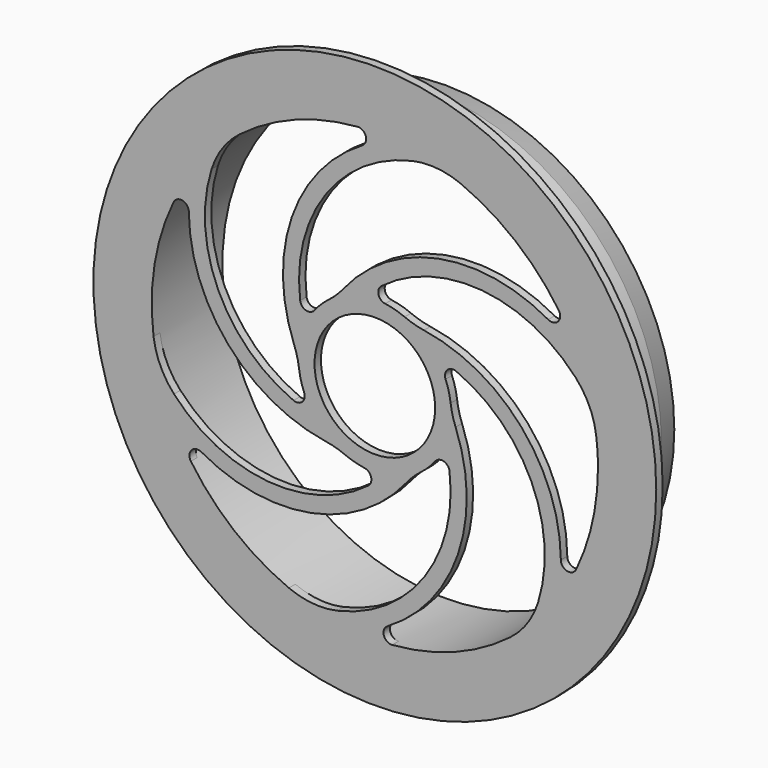
from build123d import *

# Parameters (mm, degrees)
F0_R            = 29.25
F0_R_2          = 27.75
F1_DEPTH        = 10
F2_R            = 35
F2_R_2          = 27.75
F3_DEPTH        = 1
F4_R            = 9.5
F4_R_2          = 7.5
F5_DEPTH        = 1
F7_DEPTH        = 1
F7_COPIES_COUNT = 6
F8_R            = 1
F9_T1_DEPTH     = 1
F10_SIZE2       = 0.8038475773
F10_SIZE        = 3


# Not quite as in the source:
# - a fillet or chamfer that OpenCascade refuses, or shapes differently, is made with other operations: its cross-section is extruded or revolved along the edge and cut away or added
# - a pattern or mirror of a feature is missing from the dataset's text; its kind, count and spacing are read off the source's solid


with BuildPart() as f1:
    # F0 (on Front) → F1 (new body)
    with BuildSketch(Plane.XZ):
        Circle(F0_R)
        Circle(F0_R_2, mode=Mode.SUBTRACT)
    extrude(amount=-F1_DEPTH)

    # F2 (on face) → F3 (join)
    with BuildSketch(Plane.XZ):
        Circle(F2_R)
        Circle(F2_R_2, mode=Mode.SUBTRACT)
    extrude(amount=F3_DEPTH)



with BuildPart() as f5:
    # F4 (on face) → F5 (new body)
    with BuildSketch(Plane.XZ.offset(1)):
        Circle(F4_R)
        Circle(F4_R_2, mode=Mode.SUBTRACT)
    extrude(amount=-F5_DEPTH)


with BuildPart() as f1_1:
    add(f1.part)

    add(f5.part)  # F7 merges F5
    # F6 (on face) → F7 (join)
    with BuildSketch(Plane.XZ.offset(1)):
        with BuildLine():
            ThreePointArc((8.0310171435, 26.562478492), (5.3050841985, 27.2381824219), (2.5248144723, 27.6349020603))
            ThreePointArc((2.5248144723, 27.6349020603), (-9.7684943804, 16.550468737), (-9.5, 0))
            Line((-9.5, 0), (-8.1966003247, 2.0236510077))
            ThreePointArc((-8.1966003247, 2.0236510077), (-6.4433975316, 18.4993570083), (8.0310171435, 26.562478492))
        make_face()
    f7 = extrude(amount=-F7_DEPTH)

    # F7_copies: F7 ×6 about axis
    f7_copies_axis = Axis((0, 0, 0), (0, 1, 0))
    for i in range(1, F7_COPIES_COUNT):
        add(f7.rotate(f7_copies_axis, i * 360 / F7_COPIES_COUNT))

    # F8
    f8_edges = [f1_1.edges().sort_by_distance(p)[0] for p in [
        (-8.754714, -0.5, 3.688493),
        (27.75, -0.5, 0),
        (25.194934, -0.5, 11.630898),
        (-1.183028, -0.5, 9.426051),
        (22.67012, -0.5, -16.004005),
        (7.571686, -0.5, 5.737558),
        (-2.524814, -0.5, -27.634902),
        (8.754714, -0.5, -3.688493),
        (-25.194934, -0.5, -11.630898),
        (1.183028, -0.5, -9.426051),
        (-7.571686, -0.5, -5.737558),
        (2.524814, -0.5, 27.634902),
        (-22.67012, -0.5, 16.004005),
    ]]
    fillet(f8_edges, radius=F8_R)

    # F9: fillet of radius 10 on 13 edges, made by hand

    # F9_s2 → F9_t1 (join)
    with BuildSketch(Plane.XZ):
        with BuildLine():
            ThreePointArc((-10.0443554907, 1.2572455392), (-9.6598633969, 0.0635185967), (-9.4278081059, -1.1689458148))
            ThreePointArc((-9.4278081059, -1.1689458148), (-9.4819348502, -0.5855864555), (-9.5, 0))
            ThreePointArc((-9.5, 0), (-9.7829463254, 0.6239602471), (-10.0443554907, 1.2572455392))
        make_face()
        with BuildLine():
            ThreePointArc((-5.7262408242, 7.5802484143), (-4.7749229801, 8.3974463971), (-3.9333711696, 9.3272897892))
            ThreePointArc((-3.9333711696, 9.3272897892), (-4.3511077378, 8.7842601652), (-4.75, 8.227241336))
            ThreePointArc((-4.75, 8.227241336), (-5.2481001717, 7.9188032295), (-5.7262408242, 7.5802484143))
        make_face()
        with BuildLine():
            ThreePointArc((3.7015672817, 8.7491942291), (4.8849404167, 8.3339278004), (6.1109843211, 8.07004425))
            ThreePointArc((6.1109843211, 8.07004425), (5.4318385876, 8.1602999181), (4.75, 8.227241336))
            ThreePointArc((4.75, 8.227241336), (4.2338346785, 8.504389685), (3.7015672817, 8.7491942291))
        make_face()
        with BuildLine():
            ThreePointArc((24.9752483793, 9.0272396117), (26.6725343636, 6.4844949216), (27.5222768848, 3.5477845309))
            ThreePointArc((27.5222768848, 3.5477845309), (27.3061437195, 4.9433809452), (27.0192897334, 6.3261743815))
            ThreePointArc((27.0192897334, 6.3261743815), (26.0609474008, 7.7248958252), (24.9752483793, 9.0272396117))
        make_face()
        with BuildLine():
            ThreePointArc((20.3054430194, -17.1155797565), (18.9520045147, -19.8568448814), (16.8336099733, -22.0610986868))
            ThreePointArc((16.8336099733, -22.0610986868), (17.9341653389, -21.1761236679), (18.9882725898, -20.2363041106))
            ThreePointArc((18.9882725898, -20.2363041106), (19.7204297267, -18.7069945832), (20.3054430194, -17.1155797565))
        make_face()
        with BuildLine():
            ThreePointArc((9.4278081059, 1.1689458148), (9.6598633969, -0.0635185967), (10.0443554907, -1.2572455392))
            ThreePointArc((10.0443554907, -1.2572455392), (9.7829463254, -0.6239602471), (9.5, 0))
            ThreePointArc((9.5, 0), (9.4819348502, 0.5855864555), (9.4278081059, 1.1689458148))
        make_face()
        with BuildLine():
            ThreePointArc((4.6698053599, 26.1428193681), (7.720529849, 26.341339803), (10.6886669115, 25.6088832177))
            ThreePointArc((10.6886669115, 25.6088832177), (9.3719783806, 26.1195046131), (8.0310171435, 26.562478492))
            ThreePointArc((8.0310171435, 26.562478492), (6.3405176742, 26.4318904084), (4.6698053599, 26.1428193681))
        make_face()
        with BuildLine():
            ThreePointArc((-4.6698053599, -26.1428193681), (-7.720529849, -26.341339803), (-10.6886669115, -25.6088832177))
            ThreePointArc((-10.6886669115, -25.6088832177), (-9.3719783806, -26.1195046131), (-8.0310171435, -26.562478492))
            ThreePointArc((-8.0310171435, -26.562478492), (-6.3405176742, -26.4318904084), (-4.6698053599, -26.1428193681))
        make_face()
        with BuildLine():
            ThreePointArc((5.7262408242, -7.5802484143), (4.7749229801, -8.3974463971), (3.9333711696, -9.3272897892))
            ThreePointArc((3.9333711696, -9.3272897892), (4.3511077378, -8.7842601652), (4.75, -8.227241336))
            ThreePointArc((4.75, -8.227241336), (5.2481001717, -7.9188032295), (5.7262408242, -7.5802484143))
        make_face()
        with BuildLine():
            ThreePointArc((-20.3054430194, 17.1155797565), (-18.9520045147, 19.8568448814), (-16.8336099733, 22.0610986868))
            ThreePointArc((-16.8336099733, 22.0610986868), (-17.9341653389, 21.1761236679), (-18.9882725898, 20.2363041106))
            ThreePointArc((-18.9882725898, 20.2363041106), (-19.7204297267, 18.7069945832), (-20.3054430194, 17.1155797565))
        make_face()
        with BuildLine():
            ThreePointArc((-24.9752483793, -9.0272396117), (-26.6725343636, -6.4844949216), (-27.5222768848, -3.5477845309))
            ThreePointArc((-27.5222768848, -3.5477845309), (-27.3061437195, -4.9433809452), (-27.0192897334, -6.3261743815))
            ThreePointArc((-27.0192897334, -6.3261743815), (-26.0609474008, -7.7248958252), (-24.9752483793, -9.0272396117))
        make_face()
        with BuildLine():
            ThreePointArc((-6.1109843211, -8.07004425), (-4.8849404167, -8.3339278004), (-3.7015672817, -8.7491942291))
            ThreePointArc((-3.7015672817, -8.7491942291), (-4.2338346785, -8.504389685), (-4.75, -8.227241336))
            ThreePointArc((-4.75, -8.227241336), (-5.4318385876, -8.1602999181), (-6.1109843211, -8.07004425))
        make_face()
    extrude(amount=F9_T1_DEPTH)

    # F10
    f10_edges = [f1_1.edges().sort_by_distance(p)[0] for p in [
        (-29.25, 10, 0),
    ]]
    f10_side = f1_1.faces().sort_by_distance((-29.25, 5, 0))[0]
    chamfer(f10_edges, length=F10_SIZE, length2=F10_SIZE2, reference=f10_side)


solid = f1_1.part
